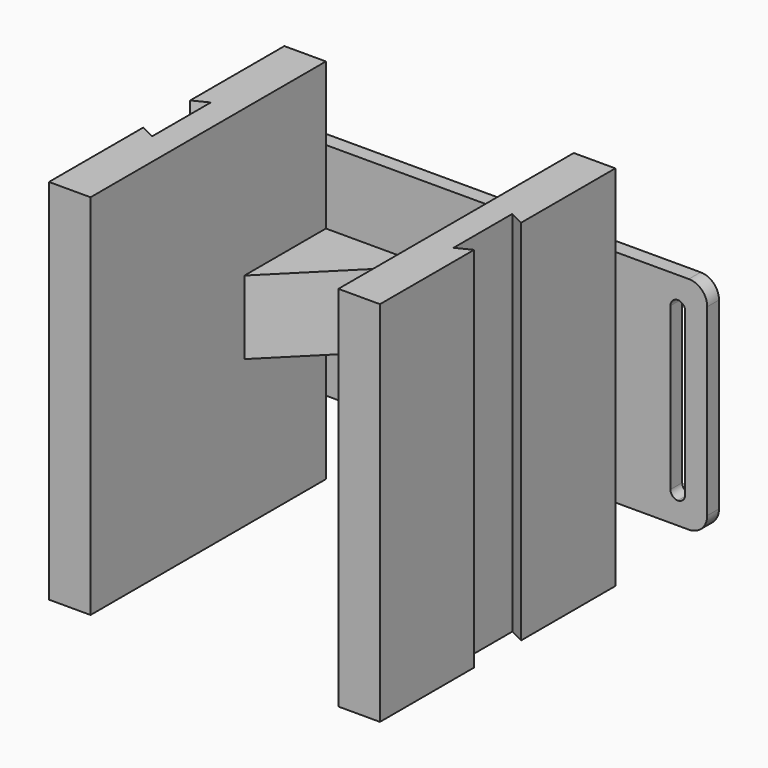
from build123d import *

# Parameters (mm, degrees)
F1_DEPTH      = 2
F2_W          = 5.6501800592
F2_H          = 10
F2_H_2        = 30
F3_DEPTH      = 40
F5_DEPTH      = 50
F7_DEPTH      = 50
F8_W          = 13.8498199408
F8_H          = 10
F9_DEPTH      = 15
F10_T4_DEPTH  = 87.150489639
F10_T10_DEPTH = 87.150489639


# Not quite as in the source:
# - a fillet or chamfer that OpenCascade refuses, or shapes differently, is made with other operations: its cross-section is extruded or revolved along the edge and cut away or added


with BuildPart() as f1:
    # F0 (on Front) → F1 (new body)
    with BuildSketch(Plane.XZ):
        with BuildLine():
            Line((32.5, 15), (-32.5, 15))
            ThreePointArc((-32.5, 15), (-34.267766953, 14.267766953), (-35, 12.5))
            Line((-35, 12.5), (-35, -12.5))
            ThreePointArc((-35, -12.5), (-34.267766953, -14.267766953), (-32.5, -15))
            Line((-32.5, -15), (32.5, -15))
            ThreePointArc((32.5, -15), (34.267766953, -14.267766953), (35, -12.5))
            Line((35, -12.5), (35, 12.5))
            ThreePointArc((35, 12.5), (34.267766953, 14.267766953), (32.5, 15))
        make_face()
        with BuildLine():
            Line((-32, -11), (-32, 11))
            ThreePointArc((-32, 11), (-31.7071067812, 11.7071067812), (-31, 12))
            ThreePointArc((-31, 12), (-30.2928932188, 11.7071067812), (-30, 11))
            Line((-30, 11), (-30, -11))
            ThreePointArc((-30, -11), (-30.2928932188, -11.7071067812), (-31, -12))
            ThreePointArc((-31, -12), (-31.7071067812, -11.7071067812), (-32, -11))
        make_face(mode=Mode.SUBTRACT)
        with BuildLine():
            Line((30, -11), (30, 11))
            ThreePointArc((30, 11), (30.2928932188, 11.7071067812), (31, 12))
            ThreePointArc((31, 12), (31.7071067812, 11.7071067812), (32, 11))
            Line((32, 11), (32, -11))
            ThreePointArc((32, -11), (31.7071067812, -11.7071067812), (31, -12))
            ThreePointArc((31, -12), (30.2928932188, -11.7071067812), (30, -11))
        make_face(mode=Mode.SUBTRACT)
    extrude(amount=F1_DEPTH)

    # F2 (on face) → F3 (join)
    with BuildSketch(Plane.XZ.offset(2)):
        with Locations((-19.6749099704, 20)):
            Rectangle(F2_W, F2_H)
        with Locations((-19.6749099704, 0)):
            Rectangle(F2_W, F2_H_2)
        with Locations((-19.6749099704, -20)):
            Rectangle(F2_W, F2_H)
        with Locations((19.6749099704, -20)):
            Rectangle(F2_W, F2_H)
        with Locations((19.6749099704, 0)):
            Rectangle(F2_W, F2_H_2)
        with Locations((19.6749099704, 20)):
            Rectangle(F2_W, F2_H)
    extrude(amount=F3_DEPTH)

    # F4 (on face) → F5 (cut, through all)
    with BuildSketch(Plane.XY.offset(25)):
        Polygon((-20.5, -17), (-22.5, -18), (-22.5, -26), (-20.5, -27), (-20.5, -26), (-20.5, -18), align=None)
    extrude(amount=-F5_DEPTH, mode=Mode.SUBTRACT)

    # F6 (on face) → F7 (cut, through all)
    with BuildSketch(Plane.XY.offset(25)):
        Polygon((22.5, -26), (22.5, -18), (20.5, -17), (20.5, -18), (20.5, -26), (20.5, -27), align=None)
    extrude(amount=-F7_DEPTH, mode=Mode.SUBTRACT)

    # F8 (on face) → F9 (join)
    with BuildSketch(Plane.XZ.offset(2)):
        with Locations((-9.9249099704, 0)):
            Rectangle(F8_W, F8_H)
        with Locations((9.9249099704, 0)):
            Rectangle(F8_W, F8_H)
    extrude(amount=F9_DEPTH)

    # F10: chamfer of 15 on 2 edges, made by hand


with BuildPart() as f10_tool2:
    # F10_s3 → F10_t4 (new body)
    with BuildSketch(Plane.XY.offset(-43.5752448195)):
        Polygon((-3, -2), (-18, -17), (-3, -17), align=None)
    extrude(amount=F10_T4_DEPTH)

    split(bisect_by=Plane.XZ.offset(2), keep=Keep.TOP)

    split(bisect_by=Plane.YZ.offset(-16.8498199408), keep=Keep.TOP)


with BuildPart() as f1_1:
    add(f1.part)

    # F10_t1: cut F10_tool2
    add(f10_tool2.part, mode=Mode.SUBTRACT)


with BuildPart() as f10_tool8:
    # F10_s9 → F10_t10 (new body)
    with BuildSketch(Plane.XY.offset(43.5752448195)):
        Polygon((3, -2), (18, -17), (3, -17), align=None)
    extrude(amount=-F10_T10_DEPTH)

    split(bisect_by=Plane.XZ.offset(2), keep=Keep.TOP)

    split(bisect_by=Plane.YZ.offset(16.8498199408), keep=Keep.BOTTOM)


with BuildPart() as f1_2:
    add(f1_1.part)

    # F10_t7: cut F10_tool8
    add(f10_tool8.part, mode=Mode.SUBTRACT)


solid = f1_2.part
